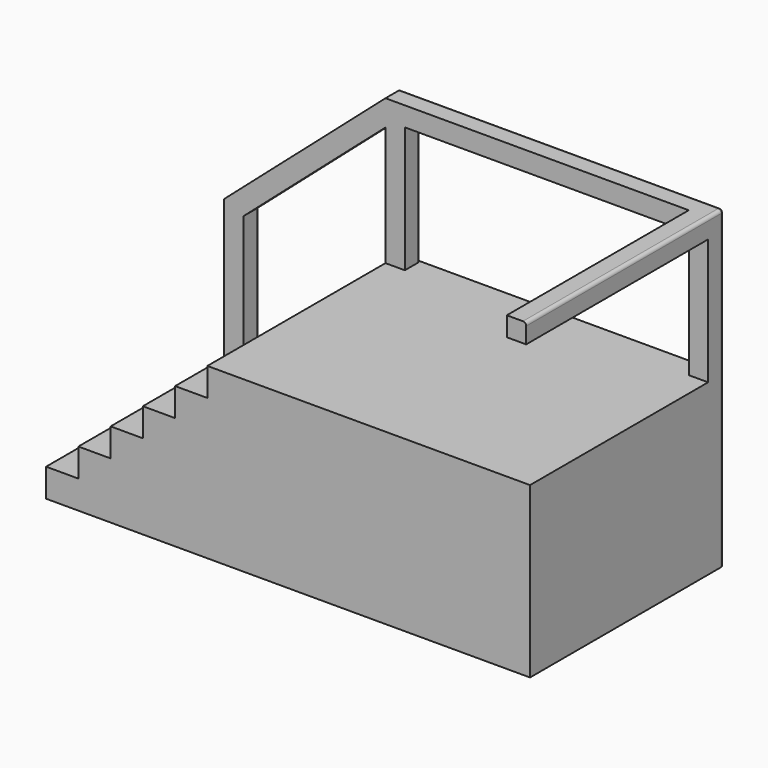
from build123d import *

# Parameters (mm, degrees)
F1_DEPTH = 15
F2_DEPTH = 1.2
F3_W     = 1.2
F3_H     = 1.2
F4_DEPTH = 14.1
F5_R     = 0.2


# Not quite as in the source:
# - a feature names something its author has since deleted; it is built from what else it names


with BuildPart() as f1:
    # F0 (on Front) → F1 (new body)
    with BuildSketch(Plane.XZ):
        Polygon((-62.2959427714, 8.75), (-63.4959427714, 8.75), (-63.4959427714, 7), (-36.9959427714, 7), (-33.4959427714, 7), (-33.4959427714, 17.5), (-34.6959427714, 17.5), (-52.2959427714, 17.5), (-53.4959427714, 17.5), (-53.4959427714, 15.75), (-55.4959427714, 15.75), (-55.4959427714, 14), (-57.4959427714, 14), (-57.4959427714, 12.25), (-59.4959427714, 12.25), (-59.4959427714, 10.5), (-61.4959427714, 10.5), (-61.4959427714, 8.75), align=None)
    extrude(amount=F1_DEPTH)

    # F0 (on Front) → F2 (join)
    with BuildSketch(Plane.XZ):
        Polygon((-61.3689829591, 19.6110898358), (-63.4959427714, 17.75), (-63.4959427714, 17.0856158867), (-63.4959427714, 16.1554781281), (-62.2959427714, 17.2054781281), (-60.5787774297, 18.7079978021), align=None)
        Polygon((-62.2959427714, 17.2054781281), (-63.4959427714, 16.1554781281), (-63.4959427714, 8.75), (-62.2959427714, 8.75), align=None)
        Polygon((-52.2959427714, 26.5), (-53.4959427714, 26.5), (-53.4959427714, 24.9054781281), (-53.4959427714, 17.5), (-52.2959427714, 17.5), (-52.2959427714, 25.3), (-52.2959427714, 26), align=None)
        Polygon((-53.4959427714, 26.5), (-61.3689829591, 19.6110898358), (-60.5787774297, 18.7079978021), (-53.4959427714, 24.9054781281), align=None)
        Polygon((-34.6959427714, 26.5), (-52.2959427714, 26.5), (-52.2959427714, 26), (-52.2959427714, 25.3), (-34.6959427714, 25.3), align=None)
        Polygon((-33.4959427714, 26.5), (-34.6959427714, 26.5), (-34.6959427714, 25.3), (-34.6959427714, 17.5), (-33.4959427714, 17.5), align=None)
    extrude(amount=F2_DEPTH)

    # F3 (on face) → F4 (join)
    with BuildSketch(Plane.XZ.offset(1.2)):
        with Locations((-34.0959427714, 25.9)):
            Rectangle(F3_W, F3_H)
    extrude(amount=F4_DEPTH)

    # F5
    f5_edges = [f1.edges().sort_by_distance(p)[0] for p in [
        (-43.495943, 0, 25.3),
        (-34.695943, 0, 21.4),
        (-52.295943, 0, 21.4),
        (-57.895943, 0, 21.055478),
        (-53.495943, 0, 20.327739),
        (-62.295943, 0, 12.977739),
        (-58.495943, 0, 22.125),
        (-43.495943, 0, 26.5),
        (-33.495943, 0, 16.75),
        (-33.495943, -7.65, 26.5),
    ]]
    fillet(f5_edges, radius=F5_R)


solid = f1.part
